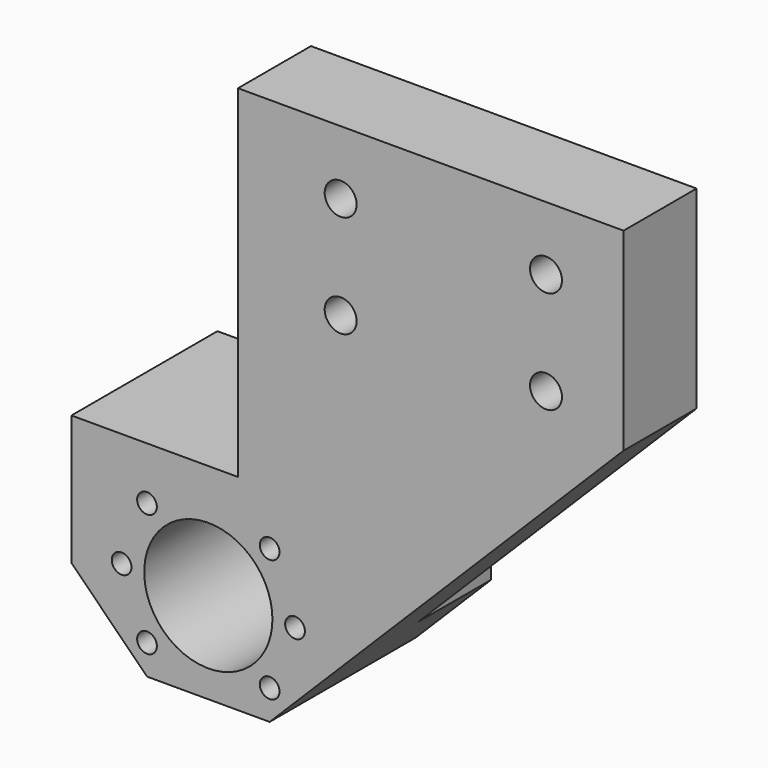
from build123d import *

# Parameters (mm, degrees)
F0_R      = 2.159
F0_R_2    = 14.05
F1_DEPTH  = 40
F2_R      = 2.159
F3_DEPTH  = 15
F5_DEPTH  = 25
F6_R      = 2.159
F7_DEPTH  = 25
F4_W      = 19
F4_H      = 20
F4_R      = 2.159
F8_DEPTH  = 25
F9_R      = 2.159
F10_DEPTH = 57.1
F11_R     = 3.5
F12_DEPTH = 20
F9_W      = 4.5
F9_H      = 20
F13_DEPTH = 25
F14_DEPTH = 50


# Not quite as in the source:
# - an extrude ends at something that could not be found from the text; its depth is read off the source's solid


with BuildPart() as f1:
    # F0 (on Front) → F1 (new body)
    with BuildSketch(Plane.XZ):
        Polygon((30, -5.94), (30, 22.5), (-30, 22.5), (-30, -5.94), (-13.44, -22.5), (13.44, -22.5), align=None)
        with Locations((-13.44, -15.94)):
            Circle(F0_R, mode=Mode.SUBTRACT)
        with Locations((-19, -2.5)):
            Circle(F0_R, mode=Mode.SUBTRACT)
        with Locations((13.44, -15.94)):
            Circle(F0_R, mode=Mode.SUBTRACT)
        with Locations((0, -2.5)):
            Circle(F0_R_2, mode=Mode.SUBTRACT)
        with Locations((19, -2.5)):
            Circle(F0_R, mode=Mode.SUBTRACT)
        with Locations((-13.44, 10.94)):
            Circle(F0_R, mode=Mode.SUBTRACT)
        with Locations((13.44, 10.94)):
            Circle(F0_R, mode=Mode.SUBTRACT)
    extrude(amount=F1_DEPTH)

    # F2 (on face) → F3 (cut)
    with BuildSketch(Plane.XY.offset(22.5)):
        with Locations((-22.5, -7)):
            Circle(F2_R)
        with Locations((22.5, -7)):
            Circle(F2_R)
        with Locations((-22.5, -33)):
            Circle(F2_R)
        with Locations((22.5, -33)):
            Circle(F2_R)
    extrude(amount=-F3_DEPTH, mode=Mode.SUBTRACT)

    # F2 (on face) → F5 (join)
    with BuildSketch(Plane.XY.offset(22.5)):
        with Locations((22.5, -33)):
            Circle(F2_R)
    extrude(amount=-F5_DEPTH)

    # F6 (on face) → F7 (join)
    with BuildSketch(Plane.XY.offset(22.5)):
        with Locations((22.5, -7)):
            Circle(F6_R)
        with Locations((22.5, -33)):
            Circle(F6_R)
        with Locations((-22.5, -7)):
            Circle(F6_R)
        with Locations((-22.5, -33)):
            Circle(F6_R)
    extrude(amount=-F7_DEPTH)

    # F4 (on face) → F8 (join)
    with BuildSketch(Plane.XY.offset(22.5)):
        with Locations((20.5, -30)):
            Rectangle(F4_W, F4_H)
        with Locations((22.5, -33)):
            Circle(F4_R, mode=Mode.SUBTRACT)
    extrude(amount=F8_DEPTH)

    # F9 (on face) → F10 (join)
    with BuildSketch(Plane.XY.offset(47.5)):
        with Locations((22.5, -33)):
            Circle(F9_R)
    extrude(amount=-F10_DEPTH)

    # F11 (on face) → F12 (join, through all)
    with BuildSketch(Plane.XZ.offset(40)):
        Polygon((11, 83.5), (11, 47.5), (30, 47.5), (30, -5.94), (91, 55.06), (91, 97.5), (11, 97.5), align=None)
        with Locations((29, 61)):
            Circle(F11_R, mode=Mode.SUBTRACT)
        with Locations((29, 83.5)):
            Circle(F11_R, mode=Mode.SUBTRACT)
        with Locations((74, 61)):
            Circle(F11_R, mode=Mode.SUBTRACT)
        with Locations((74, 83.5)):
            Circle(F11_R, mode=Mode.SUBTRACT)
    extrude(amount=-F12_DEPTH)

    # F9 (on face) → F13 (join)
    with BuildSketch(Plane.XY.offset(47.5)):
        with Locations((8.75, -30)):
            Rectangle(F9_W, F9_H)
    extrude(amount=-F13_DEPTH)

    # F9 (on face) → F14 (join, through all)
    with BuildSketch(Plane.XY.offset(47.5)):
        with Locations((8.75, -30)):
            Rectangle(F9_W, F9_H)
    extrude(amount=F14_DEPTH)


solid = f1.part
